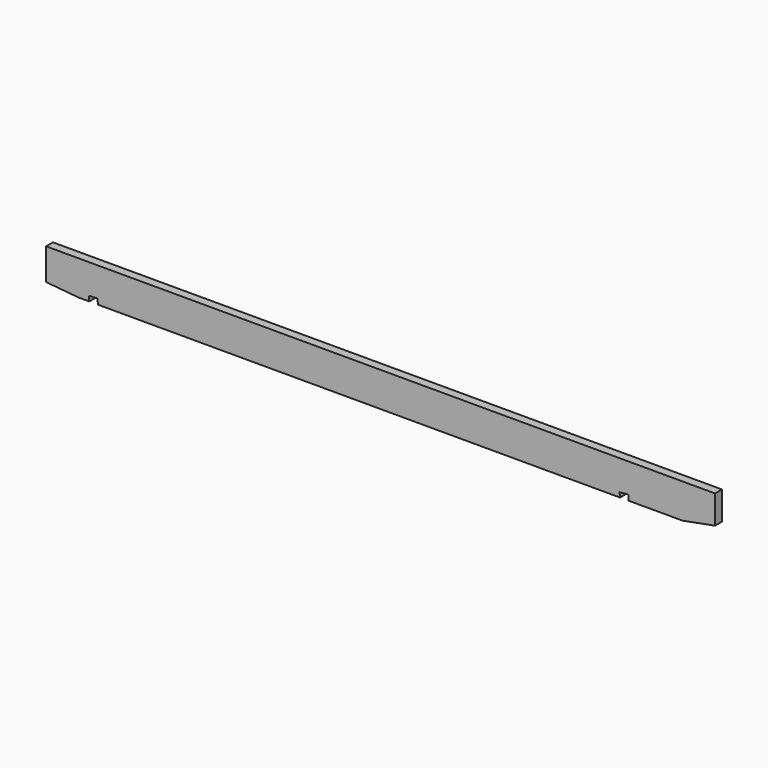
from build123d import *

# Parameters (mm, degrees)
F1_W     = 40
F1_H     = 160
F2_DEPTH = 1550
F4_DEPTH = 50


with BuildPart() as f2:
    # F1 (on Right) → F2 (new body, symmetric)
    with BuildSketch(Plane.YZ):
        Rectangle(F1_W, F1_H)
    extrude(amount=F2_DEPTH, both=True)

    # F3 (on Front) → F4 (cut, symmetric)
    with BuildSketch(Plane.XZ):
        Polygon((1823.3880364558, -300), (1823.3880364558, 0), (1400, -80), (1400, -180), (-1400, -180), (-1400, -80), (-2254.2678682115, 0), (-2254.2678682115, -300), align=None)
        Polygon((1107.8432644326, -58.8384866727), (1109.8249860087, -80), (1150, -80), (1147.6690128529, -55.1089072373), align=None)
        Polygon((-1351.3240597547, -57.380128841), (-1350, -80), (-1309.9315310961, -80), (-1311.3924116591, -55.0427199403), align=None)
    extrude(amount=F4_DEPTH, both=True, mode=Mode.SUBTRACT)


solid = f2.part
